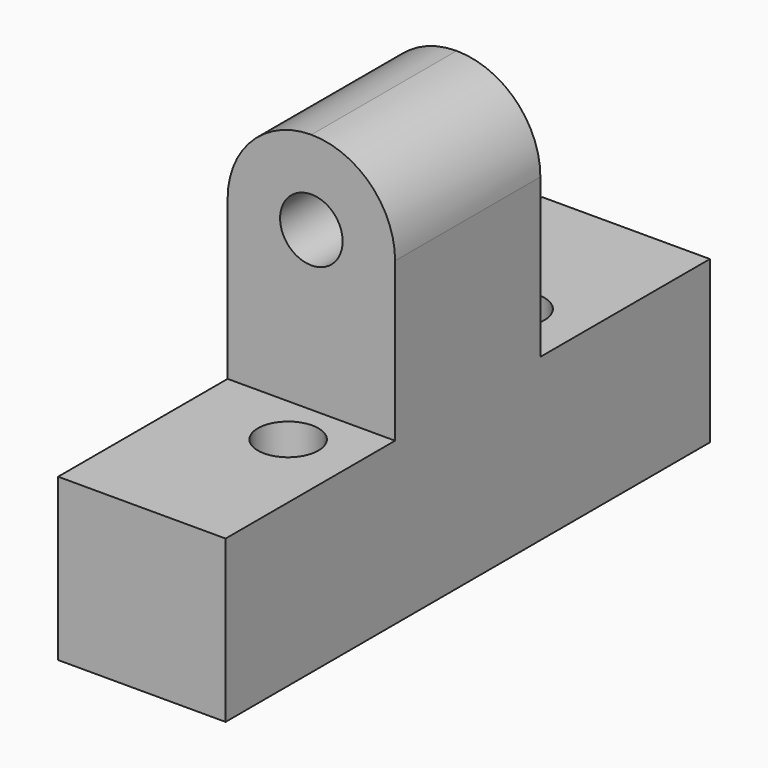
from build123d import *

# Parameters (mm, degrees)
F0_W     = 8.3
F0_H     = 30
F1_DEPTH = 8
F2_R     = 1.5
F3_DEPTH = 8.001
F4_W     = 9
F4_H     = 12
F5_DEPTH = 8.3
F6_R     = 1.55
F7_DEPTH = 19.501
F8_R     = 4.14999


# Not quite as in the source:
# - a fillet or chamfer is up to 0.001 mm smaller than in the source, because OpenCascade refuses the exact size


with BuildPart() as f1:
    # F0 (on Top) → F1 (new body)
    with BuildSketch(Plane.XY):
        Rectangle(F0_W, F0_H)
    extrude(amount=F1_DEPTH)

    # F2 (on face) → F3 (cut, through all)
    with BuildSketch(Plane.XY.offset(8)):
        with Locations((0.85, -7)):
            Circle(F2_R)
        with Locations((0.85, 7)):
            Circle(F2_R)
    extrude(amount=-F3_DEPTH, mode=Mode.SUBTRACT)

    # F4 (on face) → F5 (join, through all)
    with BuildSketch(Plane.YZ.offset(4.15)):
        with Locations((0, 14)):
            Rectangle(F4_W, F4_H)
    extrude(amount=-F5_DEPTH)

    # F6 (on face) → F7 (cut, through all)
    with BuildSketch(Plane.XZ.offset(4.5)):
        with Locations((0, 15.85)):
            Circle(F6_R)
    extrude(amount=-F7_DEPTH, mode=Mode.SUBTRACT)

    # F8 (radius 4.15 in the source; OpenCascade refuses exactly that, so slightly less here)
    f8_edges = [f1.edges().sort_by_distance(p)[0] for p in [
        (4.15, 0, 20),
        (-4.15, 0, 20),
    ]]
    fillet(f8_edges, radius=F8_R)


solid = f1.part
